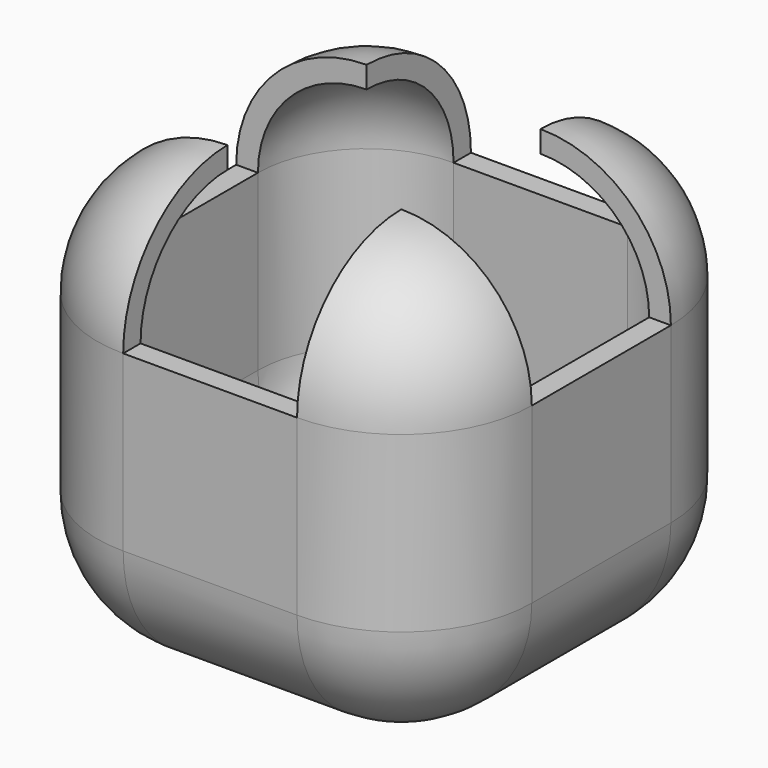
from build123d import *

# Parameters (mm, degrees)
F0_W     = 50
F0_H     = 50
F1_DEPTH = 25
F2_R     = 15
F3_R     = 15
F4_R     = 15
F5_R     = 15
F6_R     = 15
F7_T     = 2.5


# Not quite as in the source:
# - a shell that OpenCascade refuses in one call is made with other operations: the cavity is built on its own and cut out


with BuildPart() as f1:
    # F0 (on Top) → F1 (new body, symmetric)
    with BuildSketch(Plane.XY):
        Rectangle(F0_W, F0_H)
    extrude(amount=F1_DEPTH, both=True)

    # F2
    f2_edges = [f1.edges().sort_by_distance(p)[0] for p in [
        (-25, 0, 25),
    ]]
    fillet(f2_edges, radius=F2_R)

    # F3
    f3_edges = [f1.edges().sort_by_distance(p)[0] for p in [
        (7.5, -25, 25),
    ]]
    fillet(f3_edges, radius=F3_R)

    # F4
    f4_edges = [f1.edges().sort_by_distance(p)[0] for p in [
        (25, 7.5, 25),
    ]]
    fillet(f4_edges, radius=F4_R)

    # F5
    f5_edges = [f1.edges().sort_by_distance(p)[0] for p in [
        (0, 25, 25),
    ]]
    fillet(f5_edges, radius=F5_R)

    # F6
    f6_edges = [f1.edges().sort_by_distance(p)[0] for p in [
        (25, 0, -25),
    ]]
    fillet(f6_edges, radius=F6_R)

    # F7: shell of thickness 2.5, made by hand


with BuildPart() as f7_core1:
    # F7_t2: copy of F1
    add(f1.part)

    # the walls: a layer under each face that stays
    f7_faces = [f7_core1.faces().sort_by_distance(p)[0] for p in [
        (0, 0, -25),
        (20.6066017178, 0, -20.6066017178),
        (0, -20.6066017178, -20.6066017178),
        (0, 20.6066017178, -20.6066017178),
        (-20.6066017178, 0, -20.6066017178),
        (17.5, -17.5, -20.6066017178),
        (25, 0, 0),
        (17.5, 17.5, -20.6066017178),
        (-17.5, -17.5, -20.6066017178),
        (0, -25, 0),
        (0, 25, 0),
        (-17.5, 17.5, -20.6066017178),
        (-25, 0, 0),
        (20.6066017178, -20.6066017178, 0),
        (20.6066017178, 20.6066017178, 0),
        (-20.6066017178, -20.6066017178, 0),
        (-20.6066017178, 20.6066017178, 0),
        (20.6066017178, -17.5, 17.5),
        (17.5, 20.6066017178, 17.5),
        (-17.5, -20.6066017178, 17.5),
        (-17.5, 20.6066017178, 17.5),
    ]]
    thicken(f7_faces, amount=-F7_T, mode=Mode.SUBTRACT)


with BuildPart() as f1_1:
    add(f1.part)

    # what is left inside the walls is the cavity
    f7_cavity = [f7_core1.part.solids().sort_by_distance(p)[0] for p in [
        (3.333333, 20.588924, 20.588924),
    ]]
    add(f7_cavity, mode=Mode.SUBTRACT)


solid = f1_1.part
